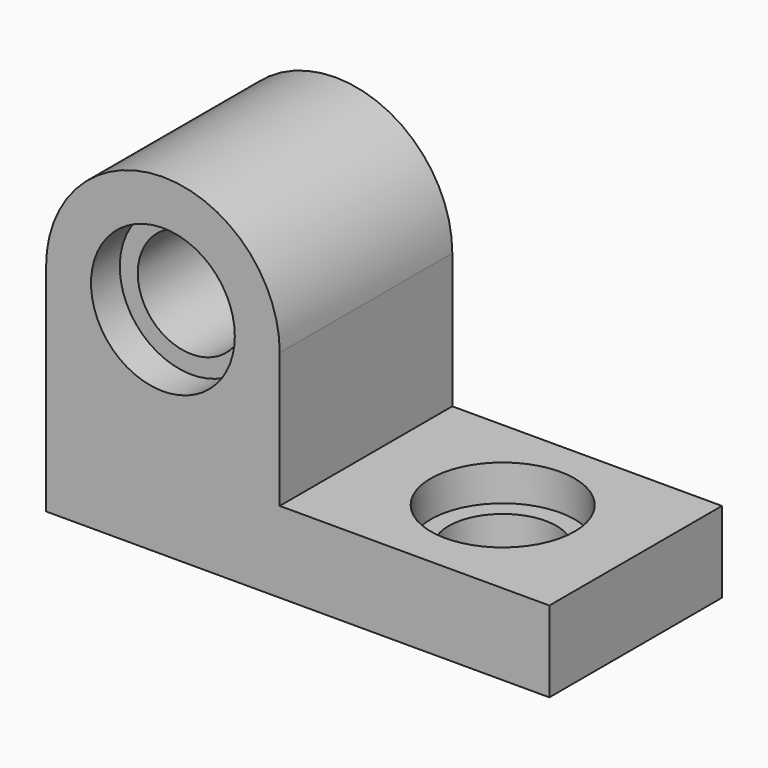
from build123d import *

# Parameters (mm, degrees)
F0_R           = 19.05
F0_W           = 95.25
F0_H           = 28.575
F1_DEPTH       = 76.2
F3_D           = 38.1
F3_CBORE_D     = 50.8
F3_CBORE_DEPTH = 12.7
F5_D           = 38.1
F5_CBORE_D     = 50.8
F5_CBORE_DEPTH = 12.7


# Not quite as in the source:
# - a length typed as a fraction of an inch, garbled in the dataset ("3 / 203.2 mm" for 3/8 in), is restored


with BuildPart() as f1:
    # F0 (on Front) → F1 (new body)
    with BuildSketch(Plane.XZ):
        with BuildLine():
            ThreePointArc((-41.275, 0), (0, -41.275), (41.275, 0))
            ThreePointArc((41.275, 0), (0, 41.275), (-41.275, 0))
        make_face()
        Circle(F0_R, mode=Mode.SUBTRACT)
        with BuildLine():
            Line((41.275, -47.625), (41.275, 0))
            ThreePointArc((41.275, 0), (0, -41.275), (-41.275, 0))
            Line((-41.275, 0), (-41.275, -76.2))
            Line((-41.275, -76.2), (41.275, -76.2))
            Line((41.275, -76.2), (41.275, -47.625))
        make_face()
        with Locations((88.9, -61.9125)):
            Rectangle(F0_W, F0_H)
        Circle(F0_R)
    extrude(amount=-F1_DEPTH)

    # F3 (through all)
    with Locations(Plane.XY.offset(-47.625)):
        with Locations((88.9528617263, 38.8567522168)):
            CounterBoreHole(F3_D / 2, F3_CBORE_D / 2, F3_CBORE_DEPTH)

    # F5 (through all)
    with Locations(Plane.XZ):
        with Locations((0, 0)):
            CounterBoreHole(F5_D / 2, F5_CBORE_D / 2, F5_CBORE_DEPTH)


solid = f1.part
